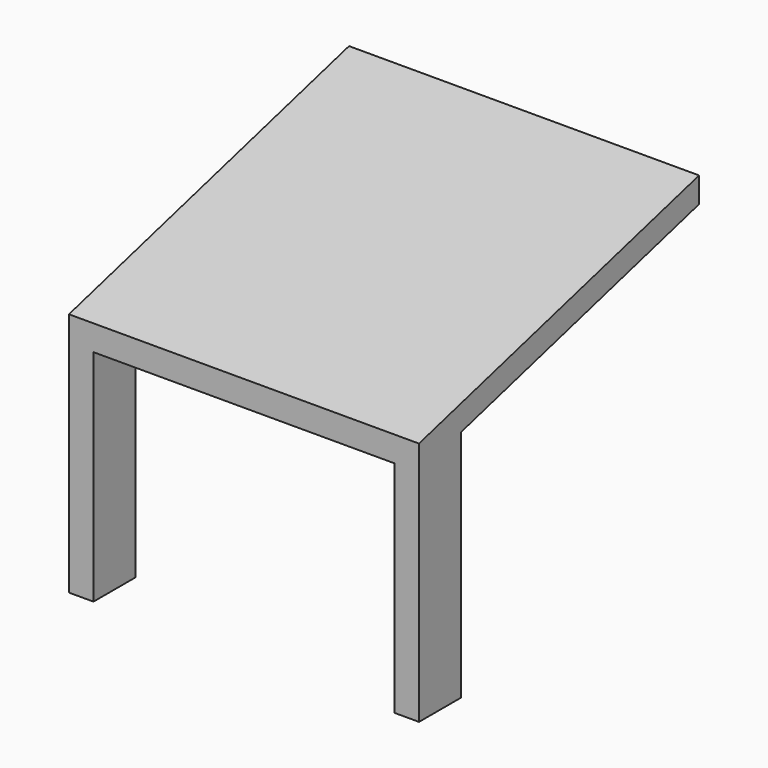
from build123d import *

# Parameters (mm, degrees)
F3_DEPTH = 250
F4_W     = 35
F4_H     = 75


# Not quite as in the source:
# - a pattern or mirror of a feature is missing from the dataset's text; its kind, count and spacing are read off the source's solid
# - the program builds the solid bodies; features that only make, move or delete a surface that nothing else refers to are left out


with BuildPart() as f3:
    # F2 (on Right) → F3 (new body, symmetric)
    with BuildSketch(Plane.YZ):
        Polygon((-500, 313.7653336856), (0, 447.7399299012), (0, 483.9745962156), (-500, 350), align=None)
    extrude(amount=F3_DEPTH, both=True)

    # F4 (on Top) → F5 (join, up to the next surface of F3)
    with BuildSketch(Plane.XY):
        with Locations((232.5, -462.5)):
            Rectangle(F4_W, F4_H)
    f5 = extrude(until=Until.NEXT)

    # F5_copies: F5 across plane
    add(f5.mirror(Plane(origin=(0, 0, 0), x_dir=(0, 0, -1), z_dir=(-1, 0, 0))))


solid = f3.part
